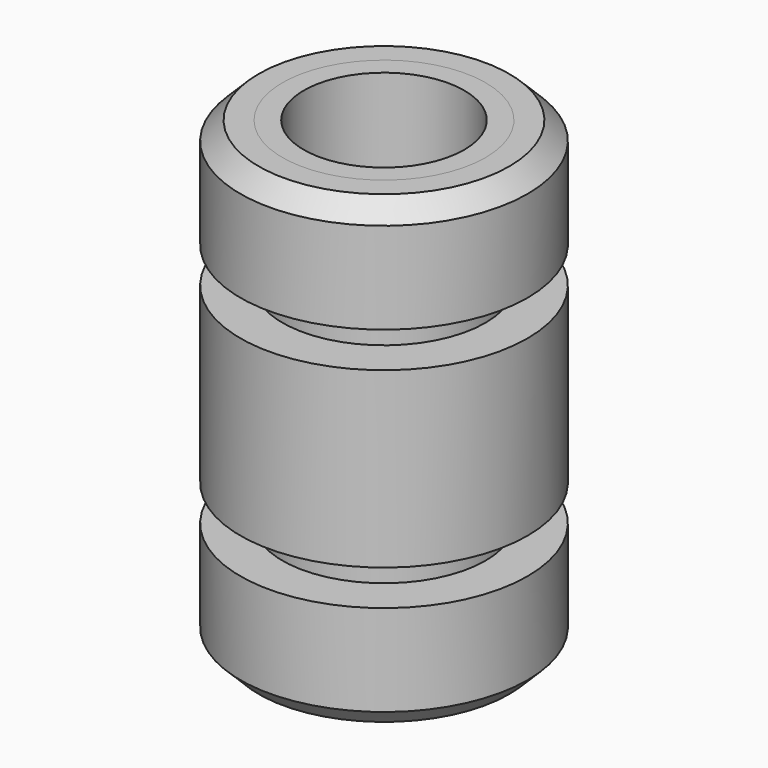
from build123d import *

# Parameters (mm, degrees)
F0_R      = 7.85
F0_R_2    = 5.55
F1_DEPTH  = 6
F2_SIZE   = 1
F5_R      = 7.85
F5_R_2    = 4.39
F6_DEPTH  = 6
F7_SIZE   = 1
F0_R_3    = 4.39
F8_DEPTH  = 25.4
F10_R     = 7.85
F10_R_2   = 4.39
F11_DEPTH = 4.75


# Not quite as in the source:
# - the program builds the solid bodies; features that only make, move or delete a surface that nothing else refers to are left out


with BuildPart() as f1:
    # F0 (on Top) → F1 (new body)
    with BuildSketch(Plane.XY):
        Circle(F0_R)
        Circle(F0_R_2, mode=Mode.SUBTRACT)
    extrude(amount=F1_DEPTH)

    # F2
    f2_edges = [f1.edges().sort_by_distance(p)[0] for p in [
        (-7.85, 0, 0),
    ]]
    chamfer(f2_edges, length=F2_SIZE)


with BuildPart() as f6:
    # F5 (on offset) → F6 (new body)
    with BuildSketch(Plane.XY.offset(25.4)):
        Circle(F5_R)
        Circle(F5_R_2, mode=Mode.SUBTRACT)
    extrude(amount=-F6_DEPTH)

    # F7
    f7_edges = [f6.edges().sort_by_distance(p)[0] for p in [
        (-7.85, 0, 25.4),
    ]]
    chamfer(f7_edges, length=F7_SIZE)


with BuildPart() as f8:
    # F0 (on Top) → F8 (new body)
    with BuildSketch(Plane.XY):
        Circle(F0_R_2)
        Circle(F0_R_3, mode=Mode.SUBTRACT)
    extrude(amount=F8_DEPTH)


with BuildPart() as f11:
    # F10 (on offset) → F11 (new body, symmetric)
    with BuildSketch(Plane.XY.offset(12.7)):
        Circle(F10_R)
        Circle(F10_R_2, mode=Mode.SUBTRACT)
    extrude(amount=F11_DEPTH, both=True)


solid = Compound([f1.part, f6.part, f8.part, f11.part])
